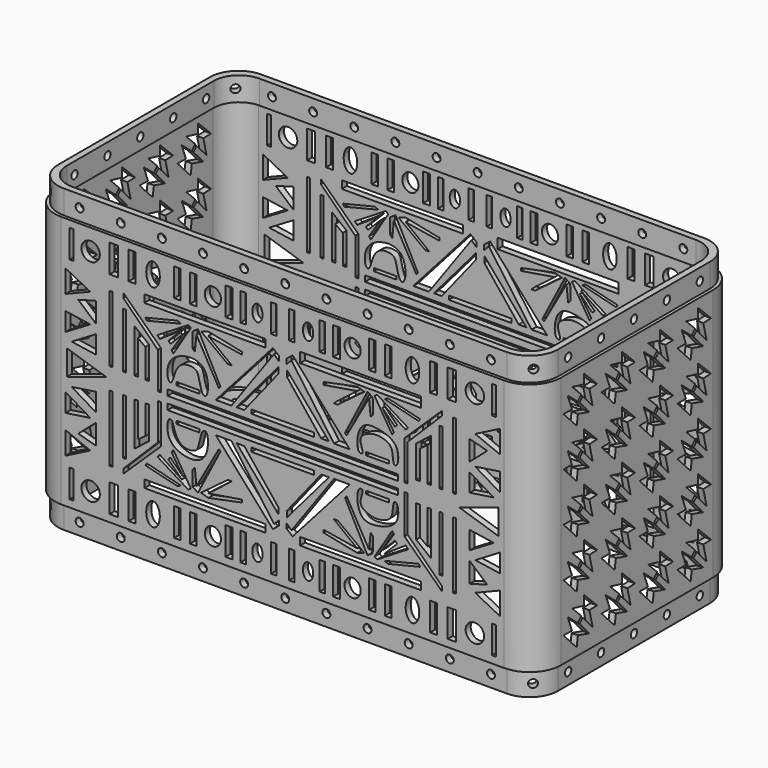
from build123d import *

# Parameters (mm, degrees)
F1_DEPTH  = 101.6
F2_T      = -2.54
F4_DEPTH  = 9.525
F6_DEPTH  = 9.525
F8_W      = 1.27
F8_H      = 26.6622491181
F8_H_2    = 22.2469121218
F8_W_2    = 48.6389496364
F8_H_3    = 3.0932202935
F8_W_3    = 9.1232359409
F8_H_4    = 1.2092068791
F8_W_4    = 12.6022342592
F8_H_5    = 1.5729144216
F8_W_5    = 46.2549291551
F8_H_6    = 2.3458786309
F8_H_7    = 4.0642395616
F8_H_8    = 0.0183284283
F8_H_9    = 3.0748918653
F8_W_6    = 1.6330480576
F8_H_10   = 11.2412478775
F8_R      = 3.7023981113
F8_W_7    = 3.2661110163
F8_W_8    = 2.7217492461
F8_W_9    = 2.6040747762
F8_W_10   = 2.5893896818
F8_W_11   = 2.1774070337
F8_W_12   = 2.7217566967
F8_W_13   = 2.1774061024
F9_DEPTH  = 127
F10_R     = 1.5875
F11_DEPTH = 127
F13_DEPTH = 228.6
F14_R     = 1.5875
F15_DEPTH = 228.6
F17_R     = 1.5875
F18_DEPTH = 50.8
F21_R     = 1.5875
F22_DEPTH = 50.8
F24_R     = 1.5875
F25_DEPTH = 76.2
F27_R     = 1.5875
F28_DEPTH = 76.2


with BuildPart() as f1:
    # F0 (on Top) → F1 (new body)
    with BuildSketch(Plane.XY):
        with BuildLine():
            Line((88.9, 50.8), (-88.9, 50.8))
            ThreePointArc((-88.9, 50.8), (-97.8802561211, 47.0802561211), (-101.6, 38.1))
            Line((-101.6, 38.1), (-101.6, -38.1))
            ThreePointArc((-101.6, -38.1), (-97.8802561211, -47.0802561211), (-88.9, -50.8))
            Line((-88.9, -50.8), (88.9, -50.8))
            ThreePointArc((88.9, -50.8), (97.8802561211, -47.0802561211), (101.6, -38.1))
            Line((101.6, -38.1), (101.6, 38.1))
            ThreePointArc((101.6, 38.1), (97.8802561211, 47.0802561211), (88.9, 50.8))
        make_face()
    extrude(amount=F1_DEPTH)

    # F2
    f2_openings = [f1.faces().sort_by_distance(p)[0] for p in [
        (0, 0, 101.6),
        (0, 0, 0),
    ]]
    offset(amount=F2_T, openings=f2_openings)

    # F3 (on face) → F4 (join)
    with BuildSketch(Plane.XY.offset(101.6)):
        with BuildLine():
            Line((-88.9, -49.53), (88.9, -49.53))
            ThreePointArc((88.9, -49.53), (96.982230509, -46.182230509), (100.33, -38.1))
            Line((100.33, -38.1), (100.33, 38.1))
            ThreePointArc((100.33, 38.1), (96.982230509, 46.182230509), (88.9, 49.53))
            Line((88.9, 49.53), (-88.9, 49.53))
            ThreePointArc((-88.9, 49.53), (-96.982230509, 46.182230509), (-100.33, 38.1))
            Line((-100.33, 38.1), (-100.33, -38.1))
            ThreePointArc((-100.33, -38.1), (-96.982230509, -46.182230509), (-88.9, -49.53))
        make_face()
        with BuildLine():
            ThreePointArc((-99.06, 38.1), (-96.0842048969, 45.2842048969), (-88.9, 48.26))
            Line((-88.9, 48.26), (88.9, 48.26))
            ThreePointArc((88.9, 48.26), (96.0842048969, 45.2842048969), (99.06, 38.1))
            Line((99.06, 38.1), (99.06, -38.1))
            ThreePointArc((99.06, -38.1), (96.0842048969, -45.2842048969), (88.9, -48.26))
            Line((88.9, -48.26), (-88.9, -48.26))
            ThreePointArc((-88.9, -48.26), (-96.0842048969, -45.2842048969), (-99.06, -38.1))
            Line((-99.06, -38.1), (-99.06, 38.1))
        make_face(mode=Mode.SUBTRACT)
        with BuildLine():
            Line((88.9, 48.26), (-88.9, 48.26))
            ThreePointArc((-88.9, 48.26), (-96.0842048969, 45.2842048969), (-99.06, 38.1))
            Line((-99.06, 38.1), (-99.06, -38.1))
            ThreePointArc((-99.06, -38.1), (-96.0842048969, -45.2842048969), (-88.9, -48.26))
            Line((-88.9, -48.26), (88.9, -48.26))
            ThreePointArc((88.9, -48.26), (96.0842048969, -45.2842048969), (99.06, -38.1))
            Line((99.06, -38.1), (99.06, 38.1))
            ThreePointArc((99.06, 38.1), (96.0842048969, 45.2842048969), (88.9, 48.26))
        make_face()
        with BuildLine():
            ThreePointArc((-97.79, 36.83), (-94.8142048969, 44.0142048969), (-87.63, 46.99))
            Line((-87.63, 46.99), (87.63, 46.99))
            ThreePointArc((87.63, 46.99), (94.8142048969, 44.0142048969), (97.79, 36.83))
            Line((97.79, 36.83), (97.79, -36.83))
            ThreePointArc((97.79, -36.83), (94.8142048969, -44.0142048969), (87.63, -46.99))
            Line((87.63, -46.99), (-87.63, -46.99))
            ThreePointArc((-87.63, -46.99), (-94.8142048969, -44.0142048969), (-97.79, -36.83))
            Line((-97.79, -36.83), (-97.79, 36.83))
        make_face(mode=Mode.SUBTRACT)
    extrude(amount=F4_DEPTH)

    # F5 (on Top) → F6 (join)
    with BuildSketch(Plane.XY):
        with BuildLine():
            Line((88.9, 49.53), (-88.9, 49.53))
            ThreePointArc((-88.9, 49.53), (-96.982230509, 46.182230509), (-100.33, 38.1))
            Line((-100.33, 38.1), (-100.33, -38.1))
            ThreePointArc((-100.33, -38.1), (-96.982230509, -46.182230509), (-88.9, -49.53))
            Line((-88.9, -49.53), (88.9, -49.53))
            ThreePointArc((88.9, -49.53), (96.982230509, -46.182230509), (100.33, -38.1))
            Line((100.33, -38.1), (100.33, 38.1))
            ThreePointArc((100.33, 38.1), (96.982230509, 46.182230509), (88.9, 49.53))
        make_face()
        with BuildLine():
            Line((87.63, -46.99), (-87.63, -46.99))
            ThreePointArc((-87.63, -46.99), (-94.8142048969, -44.0142048969), (-97.79, -36.83))
            Line((-97.79, -36.83), (-97.79, 36.83))
            ThreePointArc((-97.79, 36.83), (-94.8142048969, 44.0142048969), (-87.63, 46.99))
            Line((-87.63, 46.99), (87.63, 46.99))
            ThreePointArc((87.63, 46.99), (94.8142048969, 44.0142048969), (97.79, 36.83))
            Line((97.79, 36.83), (97.79, -36.83))
            ThreePointArc((97.79, -36.83), (94.8142048969, -44.0142048969), (87.63, -46.99))
        make_face(mode=Mode.SUBTRACT)
    extrude(amount=-F6_DEPTH)

    # F8 (on face) → F9 (cut)
    with BuildSketch(Plane.XZ.offset(50.8)):
        with Locations((-68.9020286703, 68.476928398)):
            Rectangle(F8_W, F8_H)
        with Locations((-63.4877477384, 66.1137998104)):
            Rectangle(F8_W, F8_H_2)
        Polygon((-59.5282502472, 72.5896432996), (-59.5282502472, 55.0722591579), (-58.1557303667, 55.0722591579), (-58.1557303667, 68.7985643744), (-55.1492646337, 66.6415765882), (-55.1492646337, 55.0068952143), (-53.5806752741, 55.0068952143), (-53.5806752741, 67.883476615), align=None)
        Polygon((-50.1429028809, 67.2847032547), (-50.1429028809, 52.5627210736), (-48.8572530448, 52.5627210736), (-48.8572530448, 68.2254508138), (-63.9233589172, 82.7843993902), (-63.9233589172, 80.9818580747), align=None)
        with Locations((-31.2301132362, 83.5803337395)):
            Rectangle(F8_W_2, F8_H_3)
        Polygon((-42.2406457365, 80.1282450557), (-55.1029518247, 76.9830867648), (-54.5800887048, 76.0679990053), (-40.8993884921, 79.4538781047), align=None)
        Polygon((-37.9368662834, 79.9399539828), (-50.3318198025, 72.3422840238), (-49.3153783607, 71.3319868494), (-40.5374765396, 77.2372558713), (-45.9055488806, 71.8365368266), (-45.039238331, 70.9754630211), (-40.0128401816, 76.0324299335), (-44.6069753195, 68.9266495444), (-43.8944920897, 67.867577076), (-36.8599989183, 79.27594897), align=None)
        Polygon((-36.1134645205, 78.3830672404), (-36.279860884, 72.3422840238), (-35.2634194421, 71.3319868494), (-34.6407592297, 77.6337906718), (-25.6241530731, 61.6211524411), (-24.9729361385, 62.2763298452), (-34.0206585824, 79.7909870744), align=None)
        Polygon((-32.7727422118, 79.3707743287), (-22.0318287611, 71.3319868494), (-20.3978791833, 71.3319868494), (-29.9133080989, 78.6741450429), (-16.3456853479, 76.4601826668), (-16.3456853479, 77.5059908628), (-29.8969931901, 80.269522965), align=None)
        with BuildLine():
            add(Edge.make_bspline(
                [(-45.6465967, 57.64246732), (-46.3949852869, 58.5152129663), (-46.8754204882, 65.0704943716), (-39.4761129722, 69.4554491147), (-29.7425350447, 68.3388211569), (-29.6427188035, 56.9346913808), (-32.7583018207, 56.9375001196), (-33.6608195324, 63.7843708703), (-35.1035222126, 65.6981368237), (-40.3177607972, 66.1274931074), (-43.3679070085, 62.1610139174), (-44.150056881, 57.2996314955), (-45.3474051799, 57.2935602133), (-45.6465967, 57.64246732)],
                knots=[0, 0, 0, 0, 0.1046718898, 0.2236520347, 0.3429708219, 0.4678825728, 0.5171800771, 0.6233463725, 0.6881859742, 0.7762207213, 0.869134302, 0.9581541697, 1, 1, 1, 1], degree=3))
        make_face()
        with Locations((-38.0687788129, 57.7265284956)):
            Rectangle(F8_W_3, F8_H_4)
        Polygon((-1.6442844644, 74.5871067047), (-1.6442844644, 76.9914814988), (-18.5382701457, 57.2290979326), (-15.4556166901, 57.2290979326), align=None)
        with Locations((-6.3011171296, 57.5891956687)):
            Rectangle(F8_W_4, F8_H_5)
        with Locations((6.3011171296, 57.5891956687)):
            Rectangle(F8_W_4, F8_H_5)
        with Locations((-23.1274645776, 53.396994248)):
            Rectangle(F8_W_5, F8_H_6)
        with Locations((23.1274645776, 53.396994248)):
            Rectangle(F8_W_5, F8_H_6)
        Polygon((1.6442844644, 74.5871067047), (15.4556166901, 57.2290979326), (18.5382701457, 57.2290979326), (1.6442844644, 76.9914814988), align=None)
        Polygon((49.3153783607, 71.3319868494), (50.3318198025, 72.3422840238), (37.9368662834, 79.9399539828), (36.8599989183, 79.27594897), (43.8944920897, 67.867577076), (44.6069753195, 68.9266495444), (40.0128401816, 76.0324299335), (45.039238331, 70.9754630211), (45.9055488806, 71.8365368266), (40.5374765396, 77.2372558713), align=None)
        Polygon((50.1429028809, 67.2847032547), (63.9233589172, 80.9818580747), (63.9233589172, 82.7843993902), (48.8572530448, 68.2254508138), (48.8572530448, 52.5627210736), (50.1429028809, 52.5627210736), align=None)
        Polygon((58.1557303667, 55.0722591579), (59.5282502472, 55.0722591579), (59.5282502472, 72.5896432996), (53.5806752741, 67.883476615), (53.5806752741, 55.0068952143), (55.1492646337, 55.0068952143), (55.1492646337, 66.6415765882), (58.1557303667, 68.7985643744), align=None)
        with Locations((31.2301132362, 83.0948241055)):
            Rectangle(F8_W_2, F8_H_7)
        with Locations((38.0687788129, 57.7265284956)):
            Rectangle(F8_W_3, F8_H_4)
        Polygon((35.2634194421, 71.3319868494), (36.279860884, 72.3422840238), (36.1134645205, 78.3830672404), (34.0206585824, 79.7909870744), (24.9729361385, 62.2763298452), (25.6241530731, 61.6211524411), (34.6407592297, 77.6337906718), align=None)
        Polygon((32.7727422118, 79.3707743287), (29.8969931901, 80.269522965), (16.3456853479, 77.5059908628), (16.3456853479, 76.4601826668), (29.9133080989, 78.6741450429), (20.3978791833, 71.3319868494), (22.0318287611, 71.3319868494), align=None)
        with Locations((63.4877477384, 66.1137998104)):
            Rectangle(F8_W, F8_H_2)
        with Locations((68.9020286703, 68.476928398)):
            Rectangle(F8_W, F8_H)
        Polygon((40.8993884921, 79.4538781047), (54.5800887048, 76.0679990053), (55.1029518247, 76.9830867648), (42.2406457365, 80.1282450557), align=None)
        with BuildLine():
            add(Edge.make_bspline(
                [(45.6465967, 57.64246732), (46.4635562257, 58.5803284783), (47.0830188738, 65.3489604803), (38.5305633944, 68.4932132602), (29.9974402873, 68.4019397724), (29.3300401803, 56.8501614014), (33.1351567804, 57.0444987502), (29.5108019941, 62.8747584858), (35.5677572547, 65.8582939635), (39.6837091755, 65.677942821), (44.6266519892, 63.8299183013), (43.9427154071, 57.1850526299), (45.319991823, 57.2675282703), (45.6465967, 57.64246732)],
                knots=[0, 0, 0, 0, 0.1027137574, 0.2221431268, 0.3325537808, 0.4551287654, 0.5035040447, 0.5937830457, 0.688394598, 0.7747824494, 0.8625292723, 0.9589369938, 1, 1, 1, 1], degree=3))
        make_face()
        Polygon((0, 44.9496615421), (-12.6022342592, 44.9496615421), (-12.6022342592, 43.3767471205), (0, 43.3767471205), (12.6022342592, 43.3767471205), (12.6022342592, 44.9496615421), align=None)
        Polygon((-1.6442844644, 24.7609185012), (-1.6442844644, 27.1652932953), (-15.4556166901, 44.5233020674), (-18.5382701457, 44.5233020674), align=None)
        Polygon((0, 49.5283450674), (-46.2549291551, 49.5283450674), (-46.2549291551, 47.1824664365), (0, 47.1824664365), (46.2549291551, 47.1824664365), (46.2549291551, 49.5283450674), align=None)
        Polygon((-48.8572530448, 33.5269491862), (-48.8572530448, 49.1896789264), (-50.1429028809, 49.1896789264), (-50.1429028809, 34.4676967453), (-63.9233589172, 20.7705419253), (-63.9233589172, 18.9680006098), align=None)
        Polygon((-53.5806752741, 33.868923385), (-53.5806752741, 46.7455047857), (-55.1492646337, 46.7455047857), (-55.1492646337, 35.1108234118), (-58.1557303667, 32.9538356256), (-58.1557303667, 46.6801408421), (-59.5282502472, 46.6801408421), (-59.5282502472, 29.1627567004), align=None)
        with Locations((-63.4877477384, 35.6386001896)):
            Rectangle(F8_W, F8_H_2)
        with Locations((-68.9020286703, 33.275471602)):
            Rectangle(F8_W, F8_H)
        Polygon((-36.1134645205, 23.3693327596), (-34.0206585824, 21.9614129256), (-24.9729361385, 39.4760701548), (-25.6241530731, 40.1312475589), (-34.6407592297, 24.1186093282), (-35.2634194421, 30.4204131506), (-36.279860884, 29.4101159762), align=None)
        Polygon((-32.7727422118, 22.3816256713), (-29.8969931901, 21.482877035), (-16.3456853479, 24.2464091372), (-16.3456853479, 25.2922173332), (-29.9133080989, 23.0782549571), (-20.3978791833, 30.4204131506), (-22.0318287611, 30.4204131506), align=None)
        Polygon((-49.3153783607, 30.4204131506), (-50.3318198025, 29.4101159762), (-37.9368662834, 21.8124460172), (-36.8599989183, 22.47645103), (-43.8944920897, 33.884822924), (-44.6069753195, 32.8257504556), (-40.0128401816, 25.7199700665), (-45.039238331, 30.7769369789), (-45.9055488806, 29.9158631734), (-40.5374765396, 24.5151441287), align=None)
        with Locations((-31.2301132362, 19.7095121931)):
            Rectangle(F8_W_2, F8_H_8)
        with Locations((-31.2301132362, 18.1629020463)):
            Rectangle(F8_W_2, F8_H_9)
        with Locations((-38.0687788129, 44.0258715044)):
            Rectangle(F8_W_3, F8_H_4)
        Polygon((-55.1029518247, 24.7693132352), (-42.2406457365, 21.6241549443), (-40.8993884921, 22.2985218953), (-54.5800887048, 25.6844009947), align=None)
        with BuildLine():
            add(Edge.make_bspline(
                [(-45.6465967, 44.10993268), (-46.3949852869, 43.2371870337), (-46.8754204882, 36.6819056284), (-39.4761129722, 32.2969508853), (-29.7425350447, 33.4135788431), (-29.6427188035, 44.8177086192), (-32.7583018207, 44.8148998804), (-33.6608195324, 37.9680291297), (-35.1035222126, 36.0542631763), (-40.3177607972, 35.6249068926), (-43.3679070085, 39.5913860826), (-44.150056881, 44.4527685045), (-45.3474051799, 44.4588397867), (-45.6465967, 44.10993268)],
                knots=[0, 0, 0, 0, 0.1046718898, 0.2236520347, 0.3429708219, 0.4678825728, 0.5171800771, 0.6233463725, 0.6881859742, 0.7762207213, 0.869134302, 0.9581541697, 1, 1, 1, 1], degree=3))
        make_face()
        Polygon((1.6442844644, 27.1652932953), (1.6442844644, 24.7609185012), (18.5382701457, 44.5233020674), (15.4556166901, 44.5233020674), align=None)
        with Locations((38.0687788129, 44.0258715044)):
            Rectangle(F8_W_3, F8_H_4)
        with Locations((63.4877477384, 35.6386001896)):
            Rectangle(F8_W, F8_H_2)
        Polygon((24.9729361385, 39.4760701548), (34.0206585824, 21.9614129256), (36.1134645205, 23.3693327596), (36.279860884, 29.4101159762), (35.2634194421, 30.4204131506), (34.6407592297, 24.1186093282), (25.6241530731, 40.1312475589), align=None)
        Polygon((40.8993884921, 22.2985218953), (42.2406457365, 21.6241549443), (55.1029518247, 24.7693132352), (54.5800887048, 25.6844009947), align=None)
        Polygon((37.9368662834, 21.8124460172), (50.3318198025, 29.4101159762), (49.3153783607, 30.4204131506), (40.5374765396, 24.5151441287), (45.9055488806, 29.9158631734), (45.039238331, 30.7769369789), (40.0128401816, 25.7199700665), (44.6069753195, 32.8257504556), (43.8944920897, 33.884822924), (36.8599989183, 22.47645103), align=None)
        with Locations((68.9020286703, 33.275471602)):
            Rectangle(F8_W, F8_H)
        Polygon((29.9133080989, 23.0782549571), (16.3456853479, 25.2922173332), (16.3456853479, 24.2464091372), (29.8969931901, 21.482877035), (32.7727422118, 22.3816256713), (22.0318287611, 30.4204131506), (20.3978791833, 30.4204131506), align=None)
        Polygon((58.1557303667, 32.9538356256), (55.1492646337, 35.1108234118), (55.1492646337, 46.7455047857), (53.5806752741, 46.7455047857), (53.5806752741, 33.868923385), (59.5282502472, 29.1627567004), (59.5282502472, 46.6801408421), (58.1557303667, 46.6801408421), align=None)
        Polygon((63.9233589172, 18.9680006098), (63.9233589172, 20.7705419253), (50.1429028809, 34.4676967453), (50.1429028809, 49.1896789264), (48.8572530448, 49.1896789264), (48.8572530448, 33.5269491862), align=None)
        with Locations((31.2301132362, 18.1629020463)):
            Rectangle(F8_W_2, F8_H_9)
        with Locations((31.2301132362, 19.7095121931)):
            Rectangle(F8_W_2, F8_H_8)
        with BuildLine():
            add(Edge.make_bspline(
                [(45.6465967, 44.10993268), (46.4635562257, 43.1720715217), (47.0830188738, 36.4034395197), (38.5305633944, 33.2591867398), (29.9974402873, 33.3504602276), (29.3300401803, 44.9022385986), (33.1351567804, 44.7079012498), (29.5108019941, 38.8776415142), (35.5677572547, 35.8941060365), (39.6837091755, 36.074457179), (44.6266519892, 37.9224816987), (43.9427154071, 44.5673473701), (45.319991823, 44.4848717297), (45.6465967, 44.10993268)],
                knots=[0, 0, 0, 0, 0.1027137574, 0.2221431268, 0.3325537808, 0.4551287654, 0.5035040447, 0.5937830457, 0.688394598, 0.7747824494, 0.8625292723, 0.9589369938, 1, 1, 1, 1], degree=3))
        make_face()
        Polygon((-3.9709969424, 82.8606635332), (-26.8742833287, 57.0920109749), (-20.5995067954, 57.0920109749), (-3.4801654983, 80.8973312378), (-1.516839955, 78.934006393), (-1.516839955, 80.8973312378), align=None)
        Polygon((1.516839955, 80.8973312378), (1.516839955, 78.934006393), (3.4801654983, 80.8973312378), (20.5995067954, 57.0920109749), (26.8742833287, 57.0920109749), (3.9709969424, 82.8606635332), align=None)
        Polygon((1.516839955, 22.818393607), (1.516839955, 20.8550687622), (3.9709969424, 18.8917364668), (26.8742833287, 44.6603890251), (20.5995067954, 44.6603890251), (3.4801654983, 20.8550687622), align=None)
        Polygon((-1.516839955, 22.818393607), (-3.4801654983, 20.8550687622), (-20.5995067954, 44.6603890251), (-26.8742833287, 44.6603890251), (-3.9709969424, 18.8917364668), (-1.516839955, 20.8550687622), align=None)
        with Locations((-84.7257450223, 8.5211573169)):
            Rectangle(F8_W_6, F8_H_10)
        with Locations((-77.1048292518, 8.5211573169)):
            Circle(F8_R)
        with Locations((-67.8508579731, 8.5211573169)):
            Rectangle(F8_W_7, F8_H_10)
        with Locations((-60.5021193624, 8.5211573169)):
            Rectangle(F8_W_8, F8_H_10)
        with BuildLine():
            add(Edge.make_bspline(
                [(-52.0646758378, 13.1481420249), (-56.7870740248, 13.1481420249), (-54.4258749313, 6.2076649629), (-52.0646758378, -0.7328120992), (-49.7034767442, 6.2076649629), (-47.3422776507, 13.1481420249), (-52.0646758378, 13.1481420249)],
                knots=[0, 0, 0, 2.0943951024, 2.0943951024, 4.1887902048, 4.1887902048, 6.2831853072, 6.2831853072, 6.2831853072], degree=2, weights=[1, 0.5, 1, 0.5, 1, 0.5, 1]))
        make_face()
        with Locations((-42.2663539648, 8.5211573169)):
            Rectangle(F8_W_9, F8_H_10)
        with Locations((-35.9620712698, 8.5211573169)):
            Rectangle(F8_W_10, F8_H_10)
        with BuildLine():
            add(Edge.make_bspline(
                [(-28.0320812017, 12.0741277933), (-33.6435658598, 12.0741277933), (-30.8378235307, 6.7446720786), (-28.0320812017, 1.415216364), (-25.2263388726, 6.7446720786), (-22.4205965436, 12.0741277933), (-28.0320812017, 12.0741277933)],
                knots=[0, 0, 0, 2.0943951024, 2.0943951024, 4.1887902048, 4.1887902048, 6.2831853072, 6.2831853072, 6.2831853072], degree=2, weights=[1, 0.5, 1, 0.5, 1, 0.5, 1]))
        make_face()
        with Locations((-3.6404510029, 8.5211573169)):
            Rectangle(F8_W_11, F8_H_10)
        with BuildLine():
            add(Edge.make_bspline(
                [(-10.1726669818, 11.7913372815), (-13.7381730329, 11.7913372815), (-11.9554200073, 6.8860673346), (-10.1726669818, 1.9807973877), (-8.3899139563, 6.8860673346), (-6.6071609308, 11.7913372815), (-10.1726669818, 11.7913372815)],
                knots=[0, 0, 0, 2.0943951024, 2.0943951024, 4.1887902048, 4.1887902048, 6.2831853072, 6.2831853072, 6.2831853072], degree=2, weights=[1, 0.5, 1, 0.5, 1, 0.5, 1]))
        make_face()
        with Locations((-21.604038775, 8.5211573169)):
            Rectangle(F8_W_12, F8_H_10)
        with Locations((-15.8883500844, 8.5211573169)):
            Rectangle(F8_W_13, F8_H_10)
        with Locations((84.7257450223, 8.5211573169)):
            Rectangle(F8_W_6, F8_H_10)
        with Locations((15.8883500844, 8.5211573169)):
            Rectangle(F8_W_13, F8_H_10)
        with Locations((35.9620712698, 8.5211573169)):
            Rectangle(F8_W_10, F8_H_10)
        with Locations((42.2663539648, 8.5211573169)):
            Rectangle(F8_W_9, F8_H_10)
        with Locations((21.604038775, 8.5211573169)):
            Rectangle(F8_W_12, F8_H_10)
        with Locations((67.8508579731, 8.5211573169)):
            Rectangle(F8_W_7, F8_H_10)
        with Locations((3.6404510029, 8.5211573169)):
            Rectangle(F8_W_11, F8_H_10)
        with Locations((60.5021193624, 8.5211573169)):
            Rectangle(F8_W_8, F8_H_10)
        with BuildLine():
            add(Edge.make_bspline(
                [(52.0646758378, 13.1481420249), (47.3422776507, 13.1481420249), (49.7034767442, 6.2076649629), (52.0646758378, -0.7328120992), (54.4258749313, 6.2076649629), (56.7870740248, 13.1481420249), (52.0646758378, 13.1481420249)],
                knots=[0, 0, 0, 2.0943951024, 2.0943951024, 4.1887902048, 4.1887902048, 6.2831853072, 6.2831853072, 6.2831853072], degree=2, weights=[1, 0.5, 1, 0.5, 1, 0.5, 1]))
        make_face()
        with BuildLine():
            add(Edge.make_bspline(
                [(10.1726669818, 11.7913372815), (6.6071609308, 11.7913372815), (8.3899139563, 6.8860673346), (10.1726669818, 1.9807973877), (11.9554200073, 6.8860673346), (13.7381730329, 11.7913372815), (10.1726669818, 11.7913372815)],
                knots=[0, 0, 0, 2.0943951024, 2.0943951024, 4.1887902048, 4.1887902048, 6.2831853072, 6.2831853072, 6.2831853072], degree=2, weights=[1, 0.5, 1, 0.5, 1, 0.5, 1]))
        make_face()
        with Locations((77.1048292518, 8.5211573169)):
            Circle(F8_R)
        with BuildLine():
            add(Edge.make_bspline(
                [(28.0320812017, 12.0741277933), (22.4205965436, 12.0741277933), (25.2263388726, 6.7446720786), (28.0320812017, 1.415216364), (30.8378235307, 6.7446720786), (33.6435658598, 12.0741277933), (28.0320812017, 12.0741277933)],
                knots=[0, 0, 0, 2.0943951024, 2.0943951024, 4.1887902048, 4.1887902048, 6.2831853072, 6.2831853072, 6.2831853072], degree=2, weights=[1, 0.5, 1, 0.5, 1, 0.5, 1]))
        make_face()
        with Locations((84.7257450223, 93.2312426831)):
            Rectangle(F8_W_6, F8_H_10)
        with Locations((3.6404510029, 93.2312426831)):
            Rectangle(F8_W_11, F8_H_10)
        with Locations((-42.2663539648, 93.2312426831)):
            Rectangle(F8_W_9, F8_H_10)
        with Locations((15.8883500844, 93.2312426831)):
            Rectangle(F8_W_13, F8_H_10)
        with Locations((42.2663539648, 93.2312426831)):
            Rectangle(F8_W_9, F8_H_10)
        with Locations((21.604038775, 93.2312426831)):
            Rectangle(F8_W_12, F8_H_10)
        with Locations((-15.8883500844, 93.2312426831)):
            Rectangle(F8_W_13, F8_H_10)
        with Locations((-60.5021193624, 93.2312426831)):
            Rectangle(F8_W_8, F8_H_10)
        with Locations((-67.8508579731, 93.2312426831)):
            Rectangle(F8_W_7, F8_H_10)
        with Locations((60.5021193624, 93.2312426831)):
            Rectangle(F8_W_8, F8_H_10)
        with Locations((67.8508579731, 93.2312426831)):
            Rectangle(F8_W_7, F8_H_10)
        with Locations((35.9620712698, 93.2312426831)):
            Rectangle(F8_W_10, F8_H_10)
        with Locations((-3.6404510029, 93.2312426831)):
            Rectangle(F8_W_11, F8_H_10)
        with Locations((-35.9620712698, 93.2312426831)):
            Rectangle(F8_W_10, F8_H_10)
        with Locations((-21.604038775, 93.2312426831)):
            Rectangle(F8_W_12, F8_H_10)
        with Locations((-84.7257450223, 93.2312426831)):
            Rectangle(F8_W_6, F8_H_10)
        with BuildLine():
            add(Edge.make_bspline(
                [(10.1726669818, 89.9610627185), (13.7381730329, 89.9610627185), (11.9554200073, 94.8663326654), (10.1726669818, 99.7716026123), (8.3899139563, 94.8663326654), (6.6071609308, 89.9610627185), (10.1726669818, 89.9610627185)],
                knots=[0, 0, 0, 2.0943951024, 2.0943951024, 4.1887902048, 4.1887902048, 6.2831853072, 6.2831853072, 6.2831853072], degree=2, weights=[1, 0.5, 1, 0.5, 1, 0.5, 1]))
        make_face()
        with BuildLine():
            add(Edge.make_bspline(
                [(-28.0320812017, 89.6782722067), (-22.4205965436, 89.6782722067), (-25.2263388726, 95.0077279214), (-28.0320812017, 100.337183636), (-30.8378235307, 95.0077279214), (-33.6435658598, 89.6782722067), (-28.0320812017, 89.6782722067)],
                knots=[0, 0, 0, 2.0943951024, 2.0943951024, 4.1887902048, 4.1887902048, 6.2831853072, 6.2831853072, 6.2831853072], degree=2, weights=[1, 0.5, 1, 0.5, 1, 0.5, 1]))
        make_face()
        with BuildLine():
            add(Edge.make_bspline(
                [(52.0646758378, 88.6042579751), (56.7870740248, 88.6042579751), (54.4258749313, 95.5447350371), (52.0646758378, 102.4852120992), (49.7034767442, 95.5447350371), (47.3422776507, 88.6042579751), (52.0646758378, 88.6042579751)],
                knots=[0, 0, 0, 2.0943951024, 2.0943951024, 4.1887902048, 4.1887902048, 6.2831853072, 6.2831853072, 6.2831853072], degree=2, weights=[1, 0.5, 1, 0.5, 1, 0.5, 1]))
        make_face()
        with Locations((77.1048292518, 93.2312426831)):
            Circle(F8_R)
        with BuildLine():
            add(Edge.make_bspline(
                [(28.0320812017, 89.6782722067), (33.6435658598, 89.6782722067), (30.8378235307, 95.0077279214), (28.0320812017, 100.337183636), (25.2263388726, 95.0077279214), (22.4205965436, 89.6782722067), (28.0320812017, 89.6782722067)],
                knots=[0, 0, 0, 2.0943951024, 2.0943951024, 4.1887902048, 4.1887902048, 6.2831853072, 6.2831853072, 6.2831853072], degree=2, weights=[1, 0.5, 1, 0.5, 1, 0.5, 1]))
        make_face()
        with BuildLine():
            add(Edge.make_bspline(
                [(-52.0646758378, 88.6042579751), (-47.3422776507, 88.6042579751), (-49.7034767442, 95.5447350371), (-52.0646758378, 102.4852120992), (-54.4258749313, 95.5447350371), (-56.7870740248, 88.6042579751), (-52.0646758378, 88.6042579751)],
                knots=[0, 0, 0, 2.0943951024, 2.0943951024, 4.1887902048, 4.1887902048, 6.2831853072, 6.2831853072, 6.2831853072], degree=2, weights=[1, 0.5, 1, 0.5, 1, 0.5, 1]))
        make_face()
        with BuildLine():
            add(Edge.make_bspline(
                [(-10.1726669818, 89.9610627185), (-6.6071609308, 89.9610627185), (-8.3899139563, 94.8663326654), (-10.1726669818, 99.7716026123), (-11.9554200073, 94.8663326654), (-13.7381730329, 89.9610627185), (-10.1726669818, 89.9610627185)],
                knots=[0, 0, 0, 2.0943951024, 2.0943951024, 4.1887902048, 4.1887902048, 6.2831853072, 6.2831853072, 6.2831853072], degree=2, weights=[1, 0.5, 1, 0.5, 1, 0.5, 1]))
        make_face()
        with Locations((-77.1048292518, 93.2312426831)):
            Circle(F8_R)
        Polygon((-77.2655457258, 78.9374113083), (-87.1297195554, 83.9744359255), (-87.1297195554, 74.9497637153), align=None)
        Polygon((-75.0258415937, 68.4268182709), (-75.0258415937, 76.4573417283), (-82.0926949382, 74.5300129056), align=None)
        Polygon((-77.2655457258, 67.3942267895), (-87.1297195554, 68.8633620739), (-87.1297195554, 61.5176968277), align=None)
        Polygon((-75.0258415937, 57.4427627866), (-75.0258415937, 64.6428851634), (-84.6945722448, 58.8827894529), align=None)
        Polygon((-86.6621136665, 55.9206530452), (-86.6621136665, 50.8762), (-86.6621136665, 45.8317469548), (-70.8759278059, 50.8762), align=None)
        Polygon((-75.0258415937, 37.1095148366), (-75.0258415937, 44.3096372134), (-84.6945722448, 42.8696105471), align=None)
        Polygon((-87.1297195554, 32.8890379261), (-77.2655457258, 34.3581732105), (-87.1297195554, 40.2347031723), align=None)
        Polygon((-87.1297195554, 17.7779640745), (-77.2655457258, 22.8149886917), (-87.1297195554, 26.8026362847), align=None)
        Polygon((-82.0926949382, 27.2223870944), (-75.0258415937, 25.2950582717), (-75.0258415937, 33.3255817291), align=None)
        Polygon((70.8759278059, 50.8762), (86.6621136665, 45.8317469548), (86.6621136665, 50.8762), (86.6621136665, 55.9206530452), align=None)
        Polygon((75.0258415937, 44.3096372134), (75.0258415937, 37.1095148366), (84.6945722448, 42.8696105471), align=None)
        Polygon((75.0258415937, 33.3255817291), (75.0258415937, 25.2950582717), (82.0926949382, 27.2223870944), align=None)
        Polygon((77.2655457258, 67.3942267895), (87.1297195554, 61.5176968277), (87.1297195554, 68.8633620739), align=None)
        Polygon((75.0258415937, 68.4268182709), (82.0926949382, 74.5300129056), (75.0258415937, 76.4573417283), align=None)
        Polygon((87.1297195554, 17.7779640745), (87.1297195554, 26.8026362847), (77.2655457258, 22.8149886917), align=None)
        Polygon((75.0258415937, 64.6428851634), (75.0258415937, 57.4427627866), (84.6945722448, 58.8827894529), align=None)
        Polygon((77.2655457258, 34.3581732105), (87.1297195554, 32.8890379261), (87.1297195554, 40.2347031723), align=None)
        Polygon((87.1297195554, 83.9744359255), (77.2655457258, 78.9374113083), (87.1297195554, 74.9497637153), align=None)
    extrude(amount=-F9_DEPTH, mode=Mode.SUBTRACT)

    # F10 (on face) → F11 (cut)
    with BuildSketch(Plane.XZ.offset(49.53)):
        with Locations((0, 106.3625)):
            Circle(F10_R)
        with Locations((-16.51, 106.3625)):
            Circle(F10_R)
        with Locations((-33.02, 106.3625)):
            Circle(F10_R)
        with Locations((-49.53, 106.3625)):
            Circle(F10_R)
        with Locations((-66.04, 106.3625)):
            Circle(F10_R)
        with Locations((-82.55, 106.3625)):
            Circle(F10_R)
        with Locations((16.51, 106.3625)):
            Circle(F10_R)
        with Locations((33.02, 106.3625)):
            Circle(F10_R)
        with Locations((49.53, 106.3625)):
            Circle(F10_R)
        with Locations((66.04, 106.3625)):
            Circle(F10_R)
        with Locations((82.55, 106.3625)):
            Circle(F10_R)
        with Locations((82.55, -4.7625)):
            Circle(F10_R)
        with Locations((66.04, -4.7625)):
            Circle(F10_R)
        with Locations((49.53, -4.7625)):
            Circle(F10_R)
        with Locations((33.02, -4.7625)):
            Circle(F10_R)
        with Locations((16.51, -4.7625)):
            Circle(F10_R)
        with Locations((0, -4.7625)):
            Circle(F10_R)
        with Locations((-16.51, -4.7625)):
            Circle(F10_R)
        with Locations((-33.02, -4.7625)):
            Circle(F10_R)
        with Locations((-49.53, -4.7625)):
            Circle(F10_R)
        with Locations((-66.04, -4.7625)):
            Circle(F10_R)
        with Locations((-82.55, -4.7625)):
            Circle(F10_R)
    extrude(amount=-F11_DEPTH, mode=Mode.SUBTRACT)

    # F12 (on face) → F13 (cut)
    with BuildSketch(Plane(origin=(-101.6, 0, 0), x_dir=(0, -1, 0), z_dir=(-1, 0, 0))):
        Polygon((-30.5271521211, 98.34882617), (-37.0560400188, 92.0305550098), (-33.1948697567, 91.8901413679), (-34.82172117, 85.1895782738), (-29.8476629601, 90.5899843302), (-28.2104499638, 89.0820249915), (-33.124666661, 83.7465897202), (-27.4382159114, 85.3612571955), (-26.8063880503, 81.3596844673), (-20.2345553491, 88.2172510028), (-24.4455895363, 88.2172510028), (-22.3133917898, 93.9260348678), (-27.3455451271, 89.7338111294), (-29.1230902076, 91.5391296148), (-24.5598908514, 96.032127738), (-30.5271521211, 94.5578664541), align=None)
        Polygon((-28.2104499638, 69.5240249915), (-33.124666661, 64.1885897202), (-27.4382159114, 65.8032571955), (-26.8063880503, 61.8016844673), (-20.2345553491, 68.6592510028), (-24.4455895363, 68.6592510028), (-22.3133917898, 74.3680348678), (-27.3455451271, 70.1758111294), (-29.1230902076, 71.9811296148), (-24.5598908514, 76.474127738), (-30.5271521211, 74.9998664541), (-30.5271521211, 78.79082617), (-37.0560400188, 72.4725550098), (-33.1948697567, 72.3321413679), (-34.82172117, 65.6315782738), (-29.8476629601, 71.0319843302), align=None)
        Polygon((-28.2104499638, 49.9660249915), (-33.124666661, 44.6305897202), (-27.4382159114, 46.2452571955), (-26.8063880503, 42.2436844673), (-20.2345553491, 49.1012510028), (-24.4455895363, 49.1012510028), (-22.3133917898, 54.8100348678), (-27.3455451271, 50.6178111294), (-29.1230902076, 52.4231296148), (-24.5598908514, 56.916127738), (-30.5271521211, 55.4418664541), (-30.5271521211, 59.23282617), (-37.0560400188, 52.9145550098), (-33.1948697567, 52.7741413679), (-34.82172117, 46.0735782738), (-29.8476629601, 51.4739843302), align=None)
        Polygon((-28.2104499638, 30.4080249915), (-33.124666661, 25.0725897202), (-27.4382159114, 26.6872571955), (-26.8063880503, 22.6856844673), (-20.2345553491, 29.5432510028), (-24.4455895363, 29.5432510028), (-22.3133917898, 35.2520348678), (-27.3455451271, 31.0598111294), (-29.1230902076, 32.8651296148), (-24.5598908514, 37.358127738), (-30.5271521211, 35.8838664541), (-30.5271521211, 39.67482617), (-37.0560400188, 33.3565550098), (-33.1948697567, 33.2161413679), (-34.82172117, 26.5155782738), (-29.8476629601, 31.9159843302), align=None)
        Polygon((-9.1604499638, 89.0820249915), (-14.074666661, 83.7465897202), (-8.3882159114, 85.3612571955), (-7.7563880503, 81.3596844673), (-1.1845553491, 88.2172510028), (-5.3955895363, 88.2172510028), (-3.2633917898, 93.9260348678), (-8.2955451271, 89.7338111294), (-10.0730902076, 91.5391296148), (-5.5098908514, 96.032127738), (-11.4771521211, 94.5578664541), (-11.4771521211, 98.34882617), (-18.0060400188, 92.0305550098), (-14.1448697567, 91.8901413679), (-15.77172117, 85.1895782738), (-10.7976629601, 90.5899843302), align=None)
        Polygon((-9.1604499638, 69.5240249915), (-14.074666661, 64.1885897202), (-8.3882159114, 65.8032571955), (-7.7563880503, 61.8016844673), (-1.1845553491, 68.6592510028), (-5.3955895363, 68.6592510028), (-3.2633917898, 74.3680348678), (-8.2955451271, 70.1758111294), (-10.0730902076, 71.9811296148), (-5.5098908514, 76.474127738), (-11.4771521211, 74.9998664541), (-11.4771521211, 78.79082617), (-18.0060400188, 72.4725550098), (-14.1448697567, 72.3321413679), (-15.77172117, 65.6315782738), (-10.7976629601, 71.0319843302), align=None)
        Polygon((-9.1604499638, 49.9660249915), (-14.074666661, 44.6305897202), (-8.3882159114, 46.2452571955), (-7.7563880503, 42.2436844673), (-1.1845553491, 49.1012510028), (-5.3955895363, 49.1012510028), (-3.2633917898, 54.8100348678), (-8.2955451271, 50.6178111294), (-10.0730902076, 52.4231296148), (-5.5098908514, 56.916127738), (-11.4771521211, 55.4418664541), (-11.4771521211, 59.23282617), (-18.0060400188, 52.9145550098), (-14.1448697567, 52.7741413679), (-15.77172117, 46.0735782738), (-10.7976629601, 51.4739843302), align=None)
        Polygon((-9.1604499638, 30.4080249915), (-14.074666661, 25.0725897202), (-8.3882159114, 26.6872571955), (-7.7563880503, 22.6856844673), (-1.1845553491, 29.5432510028), (-5.3955895363, 29.5432510028), (-3.2633917898, 35.2520348678), (-8.2955451271, 31.0598111294), (-10.0730902076, 32.8651296148), (-5.5098908514, 37.358127738), (-11.4771521211, 35.8838664541), (-11.4771521211, 39.67482617), (-18.0060400188, 33.3565550098), (-14.1448697567, 33.2161413679), (-15.77172117, 26.5155782738), (-10.7976629601, 31.9159843302), align=None)
        Polygon((9.8895500362, 89.0820249915), (4.975333339, 83.7465897202), (10.6617840886, 85.3612571955), (11.2936119497, 81.3596844673), (17.8654446509, 88.2172510028), (13.6544104637, 88.2172510028), (15.7866082102, 93.9260348678), (10.7544548729, 89.7338111294), (8.9769097924, 91.5391296148), (13.5401091486, 96.032127738), (7.5728478789, 94.5578664541), (7.5728478789, 98.34882617), (1.0439599812, 92.0305550098), (4.9051302433, 91.8901413679), (3.27827883, 85.1895782738), (8.2523370399, 90.5899843302), align=None)
        Polygon((9.8895500362, 69.5240249915), (4.975333339, 64.1885897202), (10.6617840886, 65.8032571955), (11.2936119497, 61.8016844673), (17.8654446509, 68.6592510028), (13.6544104637, 68.6592510028), (15.7866082102, 74.3680348678), (10.7544548729, 70.1758111294), (8.9769097924, 71.9811296148), (13.5401091486, 76.474127738), (7.5728478789, 74.9998664541), (7.5728478789, 78.79082617), (1.0439599812, 72.4725550098), (4.9051302433, 72.3321413679), (3.27827883, 65.6315782738), (8.2523370399, 71.0319843302), align=None)
        Polygon((9.8895500362, 49.9660249915), (4.975333339, 44.6305897202), (10.6617840886, 46.2452571955), (11.2936119497, 42.2436844673), (17.8654446509, 49.1012510028), (13.6544104637, 49.1012510028), (15.7866082102, 54.8100348678), (10.7544548729, 50.6178111294), (8.9769097924, 52.4231296148), (13.5401091486, 56.916127738), (7.5728478789, 55.4418664541), (7.5728478789, 59.23282617), (1.0439599812, 52.9145550098), (4.9051302433, 52.7741413679), (3.27827883, 46.0735782738), (8.2523370399, 51.4739843302), align=None)
        Polygon((9.8895500362, 30.4080249915), (4.975333339, 25.0725897202), (10.6617840886, 26.6872571955), (11.2936119497, 22.6856844673), (17.8654446509, 29.5432510028), (13.6544104637, 29.5432510028), (15.7866082102, 35.2520348678), (10.7544548729, 31.0598111294), (8.9769097924, 32.8651296148), (13.5401091486, 37.358127738), (7.5728478789, 35.8838664541), (7.5728478789, 39.67482617), (1.0439599812, 33.3565550098), (4.9051302433, 33.2161413679), (3.27827883, 26.5155782738), (8.2523370399, 31.9159843302), align=None)
        Polygon((28.9395500362, 89.0820249915), (24.025333339, 83.7465897202), (29.7117840886, 85.3612571955), (30.3436119497, 81.3596844673), (36.9154446509, 88.2172510028), (32.7044104637, 88.2172510028), (34.8366082102, 93.9260348678), (29.8044548729, 89.7338111294), (28.0269097924, 91.5391296148), (32.5901091486, 96.032127738), (26.6228478789, 94.5578664541), (26.6228478789, 98.34882617), (20.0939599812, 92.0305550098), (23.9551302433, 91.8901413679), (22.32827883, 85.1895782738), (27.3023370399, 90.5899843302), align=None)
        Polygon((28.9395500362, 69.5240249915), (24.025333339, 64.1885897202), (29.7117840886, 65.8032571955), (30.3436119497, 61.8016844673), (36.9154446509, 68.6592510028), (32.7044104637, 68.6592510028), (34.8366082102, 74.3680348678), (29.8044548729, 70.1758111294), (28.0269097924, 71.9811296148), (32.5901091486, 76.474127738), (26.6228478789, 74.9998664541), (26.6228478789, 78.79082617), (20.0939599812, 72.4725550098), (23.9551302433, 72.3321413679), (22.32827883, 65.6315782738), (27.3023370399, 71.0319843302), align=None)
        Polygon((28.9395500362, 49.9660249915), (24.025333339, 44.6305897202), (29.7117840886, 46.2452571955), (30.3436119497, 42.2436844673), (36.9154446509, 49.1012510028), (32.7044104637, 49.1012510028), (34.8366082102, 54.8100348678), (29.8044548729, 50.6178111294), (28.0269097924, 52.4231296148), (32.5901091486, 56.916127738), (26.6228478789, 55.4418664541), (26.6228478789, 59.23282617), (20.0939599812, 52.9145550098), (23.9551302433, 52.7741413679), (22.32827883, 46.0735782738), (27.3023370399, 51.4739843302), align=None)
        Polygon((28.9395500362, 30.4080249915), (24.025333339, 25.0725897202), (29.7117840886, 26.6872571955), (30.3436119497, 22.6856844673), (36.9154446509, 29.5432510028), (32.7044104637, 29.5432510028), (34.8366082102, 35.2520348678), (29.8044548729, 31.0598111294), (28.0269097924, 32.8651296148), (32.5901091486, 37.358127738), (26.6228478789, 35.8838664541), (26.6228478789, 39.67482617), (20.0939599812, 33.3565550098), (23.9551302433, 33.2161413679), (22.32827883, 26.5155782738), (27.3023370399, 31.9159843302), align=None)
        Polygon((-28.2104499638, 10.8500249915), (-33.124666661, 5.5145897202), (-27.4382159114, 7.1292571955), (-26.8063880503, 3.1276844673), (-20.2345553491, 9.9852510028), (-24.4455895363, 9.9852510028), (-22.3133917898, 15.6940348678), (-27.3455451271, 11.5018111294), (-29.1230902076, 13.3071296148), (-24.5598908514, 17.800127738), (-30.5271521211, 16.3258664541), (-30.5271521211, 20.11682617), (-37.0560400188, 13.7985550098), (-33.1948697567, 13.6581413679), (-34.82172117, 6.9575782738), (-29.8476629601, 12.3579843302), align=None)
        Polygon((-9.1604499638, 10.8500249915), (-14.074666661, 5.5145897202), (-8.3882159114, 7.1292571955), (-7.7563880503, 3.1276844673), (-1.1845553491, 9.9852510028), (-5.3955895363, 9.9852510028), (-3.2633917898, 15.6940348678), (-8.2955451271, 11.5018111294), (-10.0730902076, 13.3071296148), (-5.5098908514, 17.800127738), (-11.4771521211, 16.3258664541), (-11.4771521211, 20.11682617), (-18.0060400188, 13.7985550098), (-14.1448697567, 13.6581413679), (-15.77172117, 6.9575782738), (-10.7976629601, 12.3579843302), align=None)
        Polygon((9.8895500362, 10.8500249915), (4.975333339, 5.5145897202), (10.6617840886, 7.1292571955), (11.2936119497, 3.1276844673), (17.8654446509, 9.9852510028), (13.6544104637, 9.9852510028), (15.7866082102, 15.6940348678), (10.7544548729, 11.5018111294), (8.9769097924, 13.3071296148), (13.5401091486, 17.800127738), (7.5728478789, 16.3258664541), (7.5728478789, 20.11682617), (1.0439599812, 13.7985550098), (4.9051302433, 13.6581413679), (3.27827883, 6.9575782738), (8.2523370399, 12.3579843302), align=None)
        Polygon((28.9395500362, 10.8500249915), (24.025333339, 5.5145897202), (29.7117840886, 7.1292571955), (30.3436119497, 3.1276844673), (36.9154446509, 9.9852510028), (32.7044104637, 9.9852510028), (34.8366082102, 15.6940348678), (29.8044548729, 11.5018111294), (28.0269097924, 13.3071296148), (32.5901091486, 17.800127738), (26.6228478789, 16.3258664541), (26.6228478789, 20.11682617), (20.0939599812, 13.7985550098), (23.9551302433, 13.6581413679), (22.32827883, 6.9575782738), (27.3023370399, 12.3579843302), align=None)
    extrude(amount=-F13_DEPTH, mode=Mode.SUBTRACT)

    # F14 (on face) → F15 (cut)
    with BuildSketch(Plane.YZ.offset(100.33)):
        with Locations((0, 106.3625)):
            Circle(F14_R)
        with Locations((-16.51, 106.3625)):
            Circle(F14_R)
        with Locations((16.51, 106.3625)):
            Circle(F14_R)
        with Locations((-33.02, 106.3625)):
            Circle(F14_R)
        with Locations((33.02, 106.3625)):
            Circle(F14_R)
        with Locations((33.02, -4.7625)):
            Circle(F14_R)
        with Locations((16.51, -4.7625)):
            Circle(F14_R)
        with Locations((0, -4.7625)):
            Circle(F14_R)
        with Locations((-16.51, -4.7625)):
            Circle(F14_R)
        with Locations((-33.02, -4.7625)):
            Circle(F14_R)
    extrude(amount=-F15_DEPTH, mode=Mode.SUBTRACT)

    # F17 (on face) → F18 (cut)
    with BuildSketch(Plane(origin=(63.5, -63.5, 0), x_dir=(-0.7071067812, -0.7071067812, 0), z_dir=(-0.7071067812, 0.7071067812, 0))):
        with Locations((-35.7487341389, -4.7304881737)):
            Circle(F17_R)
        with Locations((-35.9213575721, 106.4095161855)):
            Circle(F17_R)
    extrude(amount=-F18_DEPTH, mode=Mode.SUBTRACT)

    # F21 (on face) → F22 (cut)
    with BuildSketch(Plane(origin=(-63.5, -63.5, 0), x_dir=(0.7071067812, -0.7071067812, 0), z_dir=(-0.7071067812, -0.7071067812, 0))):
        with Locations((-35.9600037336, -4.758330062)):
            Circle(F21_R)
        with Locations((-35.9600037336, 106.4215265214)):
            Circle(F21_R)
    extrude(amount=F22_DEPTH, mode=Mode.SUBTRACT)

    # F24 (on face) → F25 (cut)
    with BuildSketch(Plane(origin=(-62.223585695, 62.223585695, 0), x_dir=(-0.7071067812, -0.7071067812, 0), z_dir=(-0.7071067812, 0.7071067812, 0))):
        with Locations((35.9291117638, -4.7214720398)):
            Circle(F24_R)
        with Locations((35.9291117638, 106.4158603549)):
            Circle(F24_R)
    extrude(amount=F25_DEPTH, mode=Mode.SUBTRACT)

    # F27 (on face) → F28 (cut)
    with BuildSketch(Plane(origin=(62.223585695, 62.223585695, 0), x_dir=(0.7071067812, -0.7071067812, 0), z_dir=(-0.7071067812, -0.7071067812, 0))):
        with Locations((35.9206516296, 106.4431853592)):
            Circle(F27_R)
        with Locations((35.9206516296, -4.7728870995)):
            Circle(F27_R)
    extrude(amount=-F28_DEPTH, mode=Mode.SUBTRACT)


solid = f1.part
